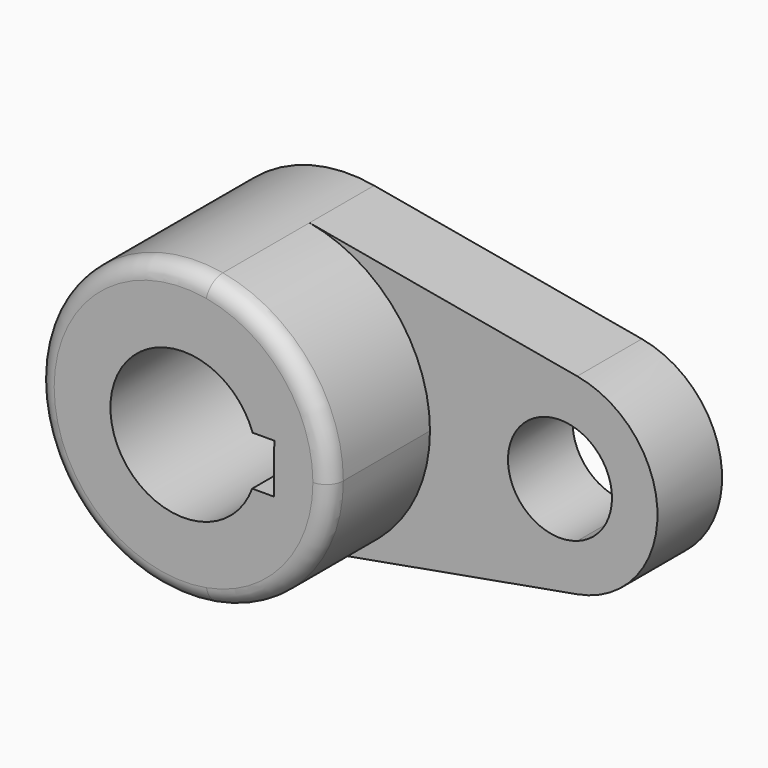
from build123d import *

# Parameters (mm, degrees)
F0_R     = 25.4
F1_DEPTH = 40.2336
F2_DEPTH = 15.7734
F3_R     = 3.302


with BuildPart() as f1:
    # F0 (on Front) → F1 (new body)
    with BuildSketch(Plane.XZ):
        with BuildLine():
            ThreePointArc((-48.9148357547, -28.1233952931), (-32.0532662831, -18.3294357754), (-25.4, 0))
            ThreePointArc((-25.4, 0), (-32.0589754437, 18.3362616868), (-48.9323529412, 28.1265414802))
            ThreePointArc((-48.9323529412, 28.1265414802), (-82.5499986144, -0.0088987403), (-48.9148357547, -28.1233952931))
        make_face()
        with Locations((-53.975, 0)):
            Circle(F0_R, mode=Mode.SUBTRACT)
        with Locations((-53.975, 0)):
            Circle(F0_R)
        with BuildLine():
            ThreePointArc((-40.5617797533, -4.9211968934), (-68.262089785, 0.1082669213), (-40.488739251, 4.717353841))
            Line((-40.488739251, 4.717353841), (-36.2469597058, 4.7305268942))
            Line((-36.2469597058, 4.7305268942), (-36.3199797533, -4.9211968934))
            Line((-36.3199797533, -4.9211968934), (-40.5617797533, -4.9211968934))
        make_face(mode=Mode.SUBTRACT)
    extrude(amount=F1_DEPTH)

    # F0 (on Front) → F2 (join)
    with BuildSketch(Plane.XZ):
        with BuildLine():
            ThreePointArc((3.3617647059, -18.7510276535), (19.05, 0), (3.3617647059, 18.7510276535))
            Line((3.3617647059, 18.7510276535), (3.3617647059, 9.5877076542))
            ThreePointArc((3.3617647059, 9.5877076542), (8.2879771178, 5.8766517077), (10.16, 0))
            ThreePointArc((10.16, 0), (8.2879771178, -5.8766517077), (3.3617647059, -9.5877076542))
            Line((3.3617647059, -9.5877076542), (3.3617647059, -18.7510276535))
        make_face()
        with BuildLine():
            ThreePointArc((-48.9323529412, 28.1265414802), (-32.0589754437, 18.3362616868), (-25.4, 0))
            ThreePointArc((-25.4, 0), (-32.0532662831, -18.3294357754), (-48.9148357547, -28.1233952931))
            Line((-48.9148357547, -28.1233952931), (3.3617647059, -18.7510276535))
            Line((3.3617647059, -18.7510276535), (3.3617647059, -9.5877076542))
            ThreePointArc((3.3617647059, -9.5877076542), (-10.16, 0), (3.3617647059, 9.5877076542))
            Line((3.3617647059, 9.5877076542), (3.3617647059, 18.7510276535))
            Line((3.3617647059, 18.7510276535), (-48.9323529412, 28.1265414802))
        make_face()
    extrude(amount=F2_DEPTH)

    # F3
    f3_edges = [f1.edges().sort_by_distance(p)[0] for p in [
        (-82.55, -40.2336, 0),
    ]]
    fillet(f3_edges, radius=F3_R)


solid = f1.part
